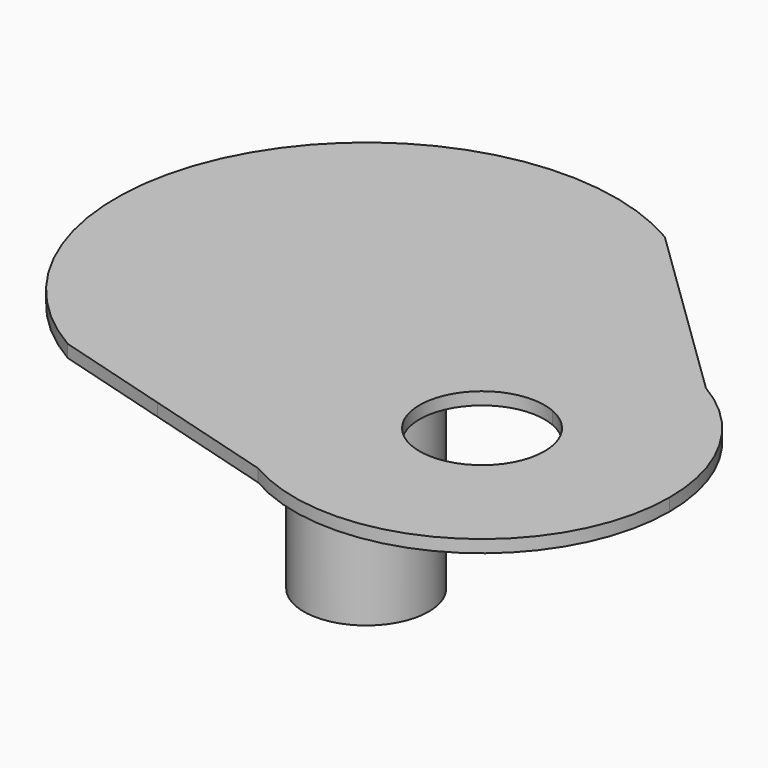
from build123d import *

# Parameters (mm, degrees)
F0_R     = 12.7
F1_DEPTH = 50.8
F3_DEPTH = 2.54
F4_R     = 1.27
F5_DEPTH = 12.7


with BuildPart() as f1:
    # F0 (on Top) → F1 (new body)
    with BuildSketch(Plane.XY):
        Circle(F0_R)
    extrude(amount=F1_DEPTH)

    # F2 (on face) → F3 (join)
    with BuildSketch(Plane.XY.offset(50.8)):
        with BuildLine():
            Line((43.181052426, 26.7588622961), (25.5085228248, 43.9312561088))
            ThreePointArc((25.5085228248, 43.9312561088), (-43.9312561088, 25.5085228248), (-25.5085228248, -43.9312561088))
            Line((-25.5085228248, -43.9312561088), (-1.833987853, -50.7668837783))
            ThreePointArc((-1.833987853, -50.7668837783), (6.0769799698, -50.4352090751), (13.8403151675, -48.87827407))
            ThreePointArc((13.8403151675, -48.87827407), (5.917077838, -28.064349578), (10.982813992, -6.3771307669))
            ThreePointArc((10.982813992, -6.3771307669), (27.3066244447, 8.7731285653), (49.3108654889, 12.2097725094))
            ThreePointArc((49.3108654889, 12.2097725094), (46.8146101479, 19.7239011532), (43.181052426, 26.7588622961))
        make_face()
        with BuildLine():
            ThreePointArc((12.7, 0), (12.2631916257, -3.3021403894), (10.982813992, -6.3771307669))
            ThreePointArc((10.982813992, -6.3771307669), (-12.2631916257, 3.3021403894), (12.7, 0))
        make_face(mode=Mode.SUBTRACT)
        with BuildLine():
            ThreePointArc((63.0626482274, 7.4399192569), (56.4166545258, 10.4876551164), (49.3108654889, 12.2097725094))
            ThreePointArc((49.3108654889, 12.2097725094), (50.4263421578, 6.150123298), (50.8, 0))
            ThreePointArc((50.8, 0), (50.3191031963, -6.9733674448), (48.8855175779, -13.8147085071))
            ThreePointArc((48.8855175779, -13.8147085071), (54.5192002119, -18.4952896423), (56.6312561088, -25.5085228248))
            ThreePointArc((56.6312561088, -25.5085228248), (49.5659896786, -36.8900770946), (36.2312911329, -35.6080544659))
            ThreePointArc((36.2312911329, -35.6080544659), (25.9001181747, -43.7015317642), (13.8403151675, -48.87827407))
            ThreePointArc((13.8403151675, -48.87827407), (18.8584152746, -54.1958484669), (24.7998639903, -58.4569649064))
            ThreePointArc((24.7998639903, -58.4569649064), (62.9405164874, -58.5275782301), (82.0312561088, -25.5085228248))
            ThreePointArc((82.0312561088, -25.5085228248), (76.9503115141, -6.4992624462), (63.0626482274, 7.4399192569))
        make_face()
        with BuildLine():
            ThreePointArc((50.8, 0), (50.4263421578, 6.150123298), (49.3108654889, 12.2097725094))
            ThreePointArc((49.3108654889, 12.2097725094), (27.3066244447, 8.7731285653), (10.982813992, -6.3771307669))
            ThreePointArc((10.982813992, -6.3771307669), (5.917077838, -28.064349578), (13.8403151675, -48.87827407))
            ThreePointArc((13.8403151675, -48.87827407), (25.9001181747, -43.7015317642), (36.2312911329, -35.6080544659))
            ThreePointArc((36.2312911329, -35.6080544659), (32.9484420816, -19.1313921186), (48.8855175779, -13.8147085071))
            ThreePointArc((48.8855175779, -13.8147085071), (50.3191031963, -6.9733674448), (50.8, 0))
        make_face()
        with BuildLine():
            ThreePointArc((12.7, 0), (-12.2631916257, 3.3021403894), (10.982813992, -6.3771307669))
            ThreePointArc((10.982813992, -6.3771307669), (12.2631916257, -3.3021403894), (12.7, 0))
        make_face()
        with BuildLine():
            Line((63.0626482274, 7.4399192569), (43.181052426, 26.7588622961))
            ThreePointArc((43.181052426, 26.7588622961), (46.8146101479, 19.7239011532), (49.3108654889, 12.2097725094))
            ThreePointArc((49.3108654889, 12.2097725094), (56.4166545258, 10.4876551164), (63.0626482274, 7.4399192569))
        make_face()
        with BuildLine():
            ThreePointArc((13.8403151675, -48.87827407), (6.0769799698, -50.4352090751), (-1.833987853, -50.7668837783))
            Line((-1.833987853, -50.7668837783), (24.7998639903, -58.4569649064))
            ThreePointArc((24.7998639903, -58.4569649064), (18.8584152746, -54.1958484669), (13.8403151675, -48.87827407))
        make_face()
    extrude(amount=F3_DEPTH)

    # F4 (on face) → F5 (cut)
    with BuildSketch(Plane(origin=(0, 0, 0), x_dir=(1, 0, 0), z_dir=(0, 0, -1))):
        Circle(F4_R)
    extrude(amount=-F5_DEPTH, mode=Mode.SUBTRACT)


solid = f1.part
